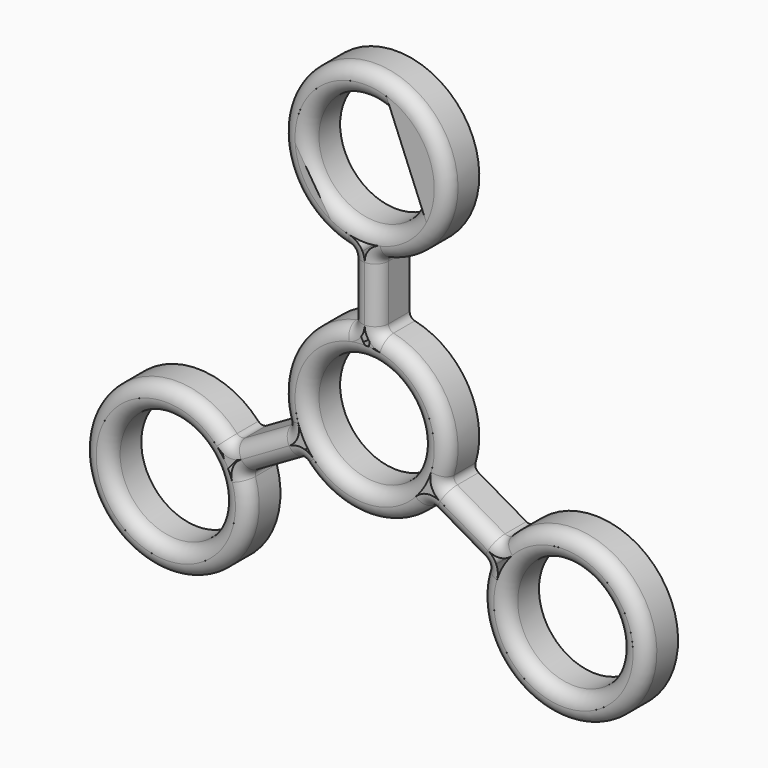
from build123d import *

# Parameters (mm, degrees)
F0_R     = 8.5
F1_DEPTH = 3
F2_R     = 1.99999


# Not quite as in the source:
# - a fillet or chamfer is up to 0.001 mm smaller than in the source, because OpenCascade refuses the exact size


with BuildPart() as f1:
    # F0 (on Front) → F1 (new body, symmetric)
    with BuildSketch(Plane.XZ):
        with BuildLine():
            ThreePointArc((12.3990131152, -4.849172483), (11.9680834103, -4.3483454973), (11.9435306622, -3.6880991474))
            ThreePointArc((11.9435306622, -3.6880991474), (10.8253175473, 6.25), (2.7777777778, 12.187450538))
            ThreePointArc((2.7777777778, 12.187450538), (2.21826404, 12.5388370166), (2, 13.1624465811))
            Line((2, 13.1624465811), (2, 21.4854950083))
            ThreePointArc((2, 21.4854950083), (2.21826404, 22.1091045727), (2.7777777778, 22.4604910513))
            ThreePointArc((2.7777777778, 22.4604910513), (0, 47.1479415894), (-2.7777777778, 22.4604910513))
            ThreePointArc((-2.7777777778, 22.4604910513), (-2.21826404, 22.1091045727), (-2, 21.4854950083))
            Line((-2, 21.4854950083), (-2, 13.1624465811))
            ThreePointArc((-2, 13.1624465811), (-2.21826404, 12.5388370166), (-2.7777777778, 12.187450538))
            ThreePointArc((-2.7777777778, 12.187450538), (-10.8253175473, 6.25), (-11.9435306622, -3.6880991474))
            ThreePointArc((-11.9435306622, -3.6880991474), (-11.9680834103, -4.3483454973), (-12.3990131152, -4.849172483))
            Line((-12.3990131152, -4.849172483), (-19.60698449, -9.0106966966))
            ThreePointArc((-19.60698449, -9.0106966966), (-20.2561782349, -9.1334792754), (-20.8402447208, -8.824619404))
            ThreePointArc((-20.8402447208, -8.824619404), (-40.8313151525, -23.5739707947), (-18.062466943, -13.6358716473))
            ThreePointArc((-18.062466943, -13.6358716473), (-18.0379141949, -12.9756252973), (-17.60698449, -12.4747983117))
            Line((-17.60698449, -12.4747983117), (-10.3990131152, -8.3132740981))
            ThreePointArc((-10.3990131152, -8.3132740981), (-9.7498193703, -8.1904915193), (-9.1657528844, -8.4993513906))
            ThreePointArc((-9.1657528844, -8.4993513906), (0, -12.5), (9.1657528844, -8.4993513906))
            ThreePointArc((9.1657528844, -8.4993513906), (9.7498193703, -8.1904915193), (10.3990131152, -8.3132740981))
            Line((10.3990131152, -8.3132740981), (17.60698449, -12.4747983117))
            ThreePointArc((17.60698449, -12.4747983117), (18.0379141949, -12.9756252973), (18.062466943, -13.6358716473))
            ThreePointArc((18.062466943, -13.6358716473), (40.8313151525, -23.5739707947), (20.8402447208, -8.824619404))
            ThreePointArc((20.8402447208, -8.824619404), (20.2561782349, -9.1334792754), (19.60698449, -9.0106966966))
            Line((19.60698449, -9.0106966966), (12.3990131152, -4.849172483))
        make_face()
        with Locations((-30.0059976052, -17.3239707947)):
            Circle(F0_R, mode=Mode.SUBTRACT)
        with Locations((30.0059976052, -17.3239707947)):
            Circle(F0_R, mode=Mode.SUBTRACT)
        Circle(F0_R, mode=Mode.SUBTRACT)
        with Locations((0, 34.6479415894)):
            Circle(F0_R, mode=Mode.SUBTRACT)
    extrude(amount=F1_DEPTH, both=True)

    # F2 (radius 2 in the source; OpenCascade refuses exactly that, so slightly less here)
    f2_edges = [f1.edges().sort_by_distance(p)[0] for p in [
        (18.037914, -3, -12.975625),
        (40.831315, -3, -23.573971),
        (20.256178, -3, -9.133479),
        (16.002999, -3, -6.929935),
        (11.968083, -3, -4.348345),
        (10.825318, -3, 6.25),
        (2.218264, -3, 12.538837),
        (2, -3, 17.323971),
        (2.218264, -3, 22.109105),
        (0, -3, 47.147942),
        (-2.218264, -3, 22.109105),
        (-2, -3, 17.323971),
        (-2.218264, -3, 12.538837),
        (-10.825318, -3, 6.25),
        (-11.968083, -3, -4.348345),
        (-16.002999, -3, -6.929935),
        (-20.256178, -3, -9.133479),
        (-40.831315, -3, -23.573971),
        (-18.037914, -3, -12.975625),
        (-14.002999, -3, -10.394036),
        (-9.749819, -3, -8.190492),
        (0, -3, -12.5),
        (9.749819, -3, -8.190492),
        (14.002999, -3, -10.394036),
        (-38.505998, -3, -17.323971),
        (21.505998, -3, -17.323971),
        (-8.5, -3, 0),
        (-8.5, -3, 34.647942),
    ]]
    fillet(f2_edges, radius=F2_R)


solid = f1.part
